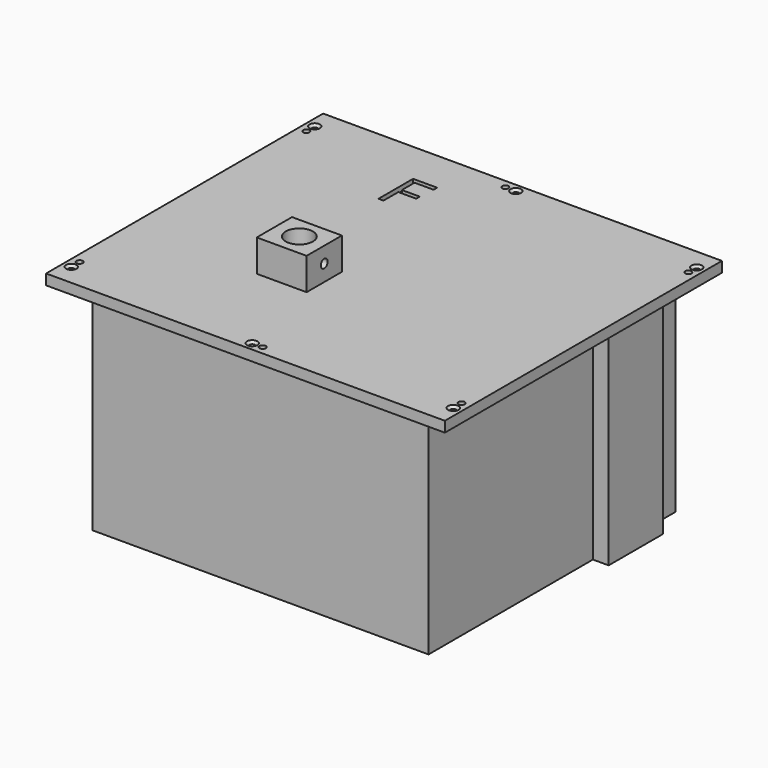
from build123d import *

# Parameters (mm, degrees)
F0_W           = 380
F0_H           = 330
F1_DEPTH       = 10
F2_W           = 15
F2_H           = 65
F3_DEPTH       = 203
F5_D           = 6
F5_DEPTH       = 10
F5_TIP         = 1.8025818571
F6_D           = 5.5
F6_DEPTH       = 10
F6_CSINK_D     = 10
F6_CSINK_ANGLE = 90
F6_TIP         = 1.6523667023
F7_W           = 47.5
F7_H           = 42
F7_R           = 13
F8_DEPTH       = 30.5
F9_TEXT_SIZE   = 57.7048812475
F10_DEPTH      = 5
F11_R          = 4.1
F12_DEPTH      = 62.5
F13_DEPTH      = 10


# Not quite as in the source:
# - Text() gives the source's letters only with a copy of the font that has no kerning and outlines rounded to 1/6400 em; it was checked with that copy


with BuildPart() as f1:
    # F0 (on Top) → F1 (new body)
    with BuildSketch(Plane.XY):
        Rectangle(F0_W, F0_H)
    extrude(amount=F1_DEPTH)

    # F2 (on face) → F3 (join)
    with BuildSketch(Plane(origin=(0, 0, 0), x_dir=(1, 0, 0), z_dir=(0, 0, -1))):
        Polygon((-160.15, -147.15), (160.15, -147.15), (160.15, -113.65), (160.15, -48.65), (160.15, 147.15), (-160.15, 147.15), align=None)
        with Locations((167.65, -81.15)):
            Rectangle(F2_W, F2_H)
    extrude(amount=F3_DEPTH)

    # F5
    with Locations(Plane.XY.offset(10)):
        with Locations((-182, 135), (-182, -135), (182, 135), (182, -135), (10, -157), (-10, 157)):
            Hole(F5_D / 2, depth=F5_DEPTH)
            with Locations((0, 0, -(F5_DEPTH + F5_TIP / 2))):  # 118° drill point
                Cone(0, F5_D / 2, F5_TIP, mode=Mode.SUBTRACT)

    # F6
    with Locations(Plane.XY.offset(10)):
        with Locations((-182, 145), (182, 145), (-182, -145), (182, -145), (0, -157), (0, 157)):
            CounterSinkHole(F6_D / 2, F6_CSINK_D / 2, depth=F6_DEPTH, counter_sink_angle=F6_CSINK_ANGLE)
            with Locations((0, 0, -(F6_DEPTH + F6_TIP / 2))):  # 118° drill point
                Cone(0, F6_D / 2, F6_TIP, mode=Mode.SUBTRACT)

    # F7 (on face) → F8 (join)
    with BuildSketch(Plane.XY.offset(10)):
        with Locations((-43.5, -46.5)):
            Rectangle(F7_W, F7_H)
        with Locations((-43.5, -46.5)):
            Circle(F7_R, mode=Mode.SUBTRACT)
    extrude(amount=F8_DEPTH)

    # F9 (on face) → F10 (cut)
    with BuildSketch(Plane.XY.offset(10)):
        with Locations((-77.71358639, 83.5087820888)):
            Text('F', F9_TEXT_SIZE, font='Open Sans', text_align=(TextAlign.LEFT, TextAlign.BOTTOM))
    extrude(amount=-F10_DEPTH, mode=Mode.SUBTRACT)

    # F11 (on face) → F12 (cut)
    with BuildSketch(Plane(origin=(-67.25, 0, 0), x_dir=(0, -1, 0), z_dir=(-1, 0, 0))):
        with Locations((46.5, 25.5)):
            Circle(F11_R)
    extrude(amount=-F12_DEPTH, mode=Mode.SUBTRACT)

    # F13 (cut): a face of the model
    f13_faces = [f1.faces().sort_by_distance(p)[0] for p in [
        (-43.5, -46.5, 10),
    ]]
    extrude(f13_faces, amount=-F13_DEPTH, mode=Mode.SUBTRACT)


solid = f1.part
